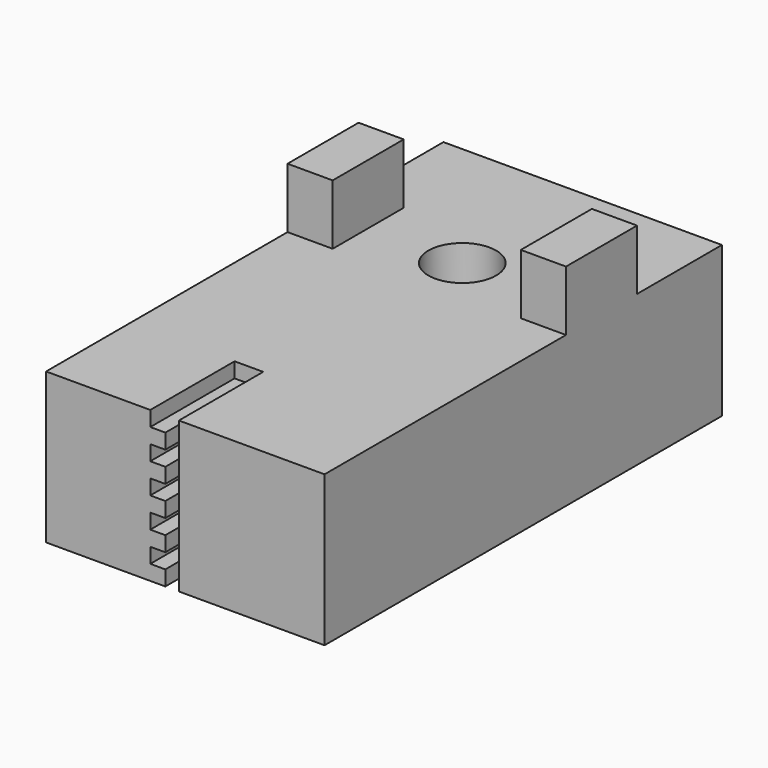
from build123d import *

# Parameters (mm, degrees)
F0_W     = 18.5
F0_H     = 13
F1_DEPTH = 10
F0_W_2   = 3
F0_H_2   = 2.95
F2_DEPTH = 14
F4_DEPTH = 7
F5_R     = 4
F5_R_2   = 2.25
F6_DEPTH = 6


# Not quite as in the source:
# - a fillet or chamfer that OpenCascade refuses, or shapes differently, is made with other operations: its cross-section is extruded or revolved along the edge and cut away or added


with BuildPart() as f1:
    # F0 (on Top) → F1 (new body)
    with BuildSketch(Plane.XY):
        with BuildLine():
            Line((-4.96357069, 33), (-4.96357069, 25.95))
            Line((-4.96357069, 25.95), (-1.96357069, 25.95))
            Line((-1.96357069, 25.95), (-1.96357069, 23))
            Line((-1.96357069, 23), (2.03642931, 23))
            ThreePointArc((2.03642931, 23), (4.28642931, 25.25), (6.53642931, 23))
            Line((6.53642931, 23), (10.53642931, 23))
            Line((10.53642931, 23), (10.53642931, 25.95))
            Line((10.53642931, 25.95), (13.53642931, 25.95))
            Line((13.53642931, 25.95), (13.53642931, 33))
            Line((13.53642931, 33), (-4.96357069, 33))
        make_face()
        with BuildLine():
            Line((-4.96357069, 20.05), (-4.96357069, 13))
            Line((-4.96357069, 13), (13.53642931, 13))
            Line((13.53642931, 13), (13.53642931, 20.05))
            Line((13.53642931, 20.05), (10.53642931, 20.05))
            Line((10.53642931, 20.05), (10.53642931, 23))
            Line((10.53642931, 23), (6.53642931, 23))
            ThreePointArc((6.53642931, 23), (4.28642931, 20.75), (2.03642931, 23))
            Line((2.03642931, 23), (-1.96357069, 23))
            Line((-1.96357069, 23), (-1.96357069, 20.05))
            Line((-1.96357069, 20.05), (-4.96357069, 20.05))
        make_face()
        with Locations((4.28642931, 6.5)):
            Rectangle(F0_W, F0_H)
    extrude(amount=F1_DEPTH)

    # F0 (on Top) → F2 (join)
    with BuildSketch(Plane.XY):
        with Locations((-3.46357069, 21.525)):
            Rectangle(F0_W_2, F0_H_2)
        with Locations((-3.46357069, 24.475)):
            Rectangle(F0_W_2, F0_H_2)
        with Locations((12.03642931, 24.475)):
            Rectangle(F0_W_2, F0_H_2)
        with Locations((12.03642931, 21.525)):
            Rectangle(F0_W_2, F0_H_2)
    extrude(amount=F2_DEPTH)

    # F3 (on face) → F4 (cut)
    with BuildSketch(Plane.XZ):
        Polygon((3.8593590405, 10), (1.9593590405, 10), (1.9593590405, 9), (2.9593590405, 9), (2.9593590405, 8), (1.9593590405, 8), (1.9593590405, 7), (2.9593590405, 7), (2.9593590405, 6), (1.9593590405, 6), (1.9593590405, 5), (2.9593590405, 5), (2.9593590405, 4), (1.9593590405, 4), (1.9593590405, 3), (2.9593590405, 3), (2.9593590405, 2), (1.9593590405, 2), (1.9593590405, 1), (2.9593590405, 1), (2.9593590405, 0), (3.8593590405, 0), align=None)
    extrude(amount=-F4_DEPTH, mode=Mode.SUBTRACT)

    # F5 (on face) → F6 (cut)
    with BuildSketch(Plane(origin=(0, 0, 0), x_dir=(1, 0, 0), z_dir=(0, 0, -1))):
        with Locations((4.28642931, -23)):
            Circle(F5_R)
        with Locations((4.28642931, -23)):
            Circle(F5_R_2, mode=Mode.SUBTRACT)
    extrude(amount=-F6_DEPTH, mode=Mode.SUBTRACT)

    # F7: fillet of radius 3 on 1 edges, made by hand

    # F7_s1 → F7_t2 (revolve)
    with BuildSketch(Plane.XZ.offset(-23)):
        with BuildLine():
            ThreePointArc((8.28642931, 3.2728219713), (7.8113055446, 4.8930071459), (6.53642931, 6))
            Line((6.53642931, 6), (8.28642931, 6))
            Line((8.28642931, 6), (8.28642931, 3.2728219713))
        make_face()
    revolve(axis=Axis((4.28642931, 23, 6), (0, 0, -1)))


solid = f1.part
